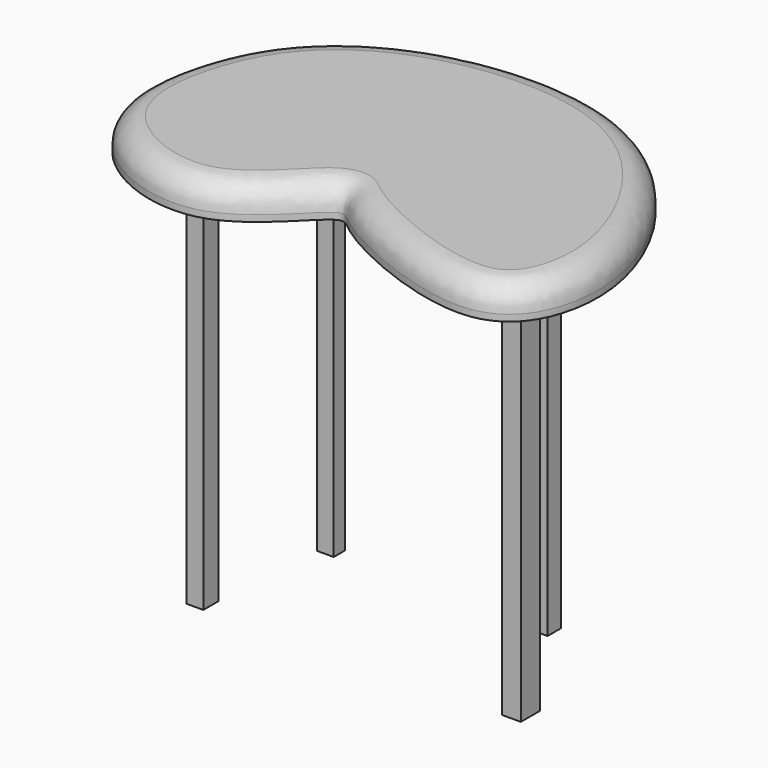
from build123d import *

# Parameters (mm, degrees)
F1_DEPTH = 6.35
F2_R     = 5.08
F3_W     = 3.2562203705
F3_H     = 3.7213950418
F3_W_2   = 3.7213936448
F3_H_2   = 4.6517443843
F3_H_3   = 2.791043371
F3_W_3   = 3.2562240958
F3_H_4   = 3.2562203705
F4_DEPTH = 76.2


with BuildPart() as f1:
    # F0 (on Top) → F1 (new body)
    with BuildSketch(Plane.XY):
        with BuildLine():
            add(Edge.make_bspline(
                [(0, -6.0472674668), (-2.7942810248, -7.2532823319), (-15.159403315, -25.6842774883), (-47.9393784632, -11.7743783852), (-44.6845666377, 15.4614801681), (-34.6336399208, 31.631588662), (-15.6821885669, 42.2121533956), (10.6018744389, 44.0959391337), (31.4662127724, 34.6879526205), (45.0578731665, 15.1655328703), (49.4110798899, -5.512282388), (38.531823197, -25.2385634551), (3.7930302773, -9.5252248366), (1.3377787026, -5.4698806588), (0, -6.0472674668)],
                knots=[0, 0, 0, 0, 0.08279823, 0.178919396, 0.2677776921, 0.3467750881, 0.4301683374, 0.5229381413, 0.6088051336, 0.6966423299, 0.7795905132, 0.854013421, 0.9603598537, 1, 1, 1, 1], degree=3))
        make_face()
    extrude(amount=F1_DEPTH)

    # F2
    f2_edges = [f1.edges().sort_by_distance(p)[0] for p in [
        (1.936589, 42.808202, 6.35),
    ]]
    fillet(f2_edges, radius=F2_R)

    # F3 (on Top) → F4 (join)
    with BuildSketch(Plane.XY):
        with Locations((-28.1430520117, -4.1865697131)):
            Rectangle(F3_W, F3_H)
        with Locations((33.0273844302, -2.3258721922)):
            Rectangle(F3_W_2, F3_H_2)
        with Locations((-23.4913080931, 21.6306112707)):
            Rectangle(F3_W, F3_H_3)
        with Locations((18.6069756746, 21.8631979078)):
            Rectangle(F3_W_3, F3_H_4)
    extrude(amount=-F4_DEPTH)


solid = f1.part
